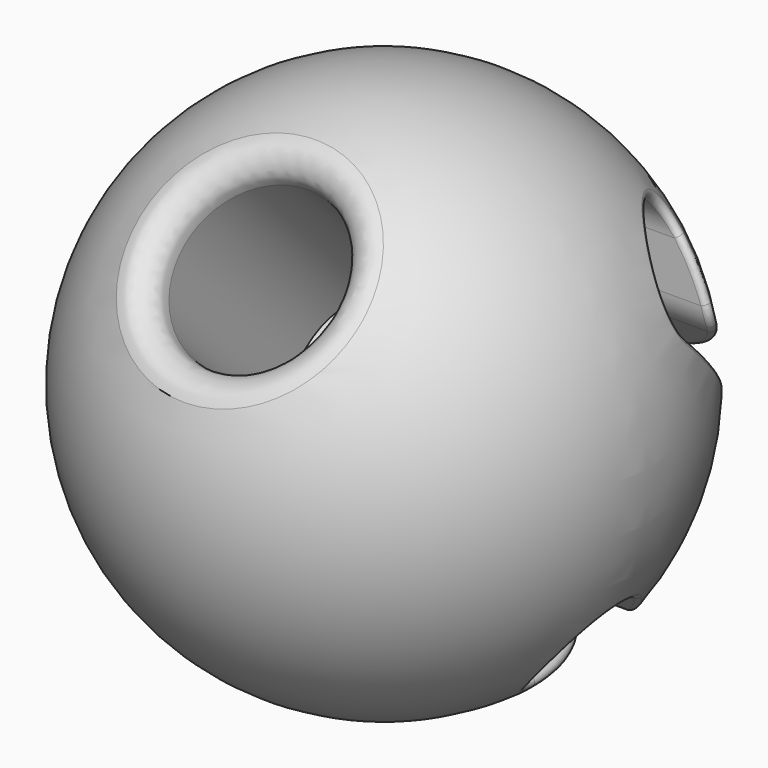
from build123d import *

# Parameters (mm, degrees)
F5_R     = 1
F6_DEPTH = 4
F8_DEPTH = 12.5
F9_R     = 0.3
F10_R    = 0.06


with BuildPart() as f2:
    # F0 (on Front) → F2 (revolve)
    with BuildSketch(Plane.XZ):
        with BuildLine():
            ThreePointArc((0, -3.25), (3.25, 0), (0, 3.25))
            Line((0, 3.25), (0, -3.25))
        make_face()
    revolve(axis=Axis((0, 0, 0.1662829891), (0, 0, 1)))

    # F5 (on face) → F6 (cut)
    with BuildSketch(Plane(origin=(0, -2.8284271247, 2.8284271247), x_dir=(1, 0, 0), z_dir=(0, -0.7071067812, 0.7071067812))):
        Circle(F5_R)
    extrude(amount=-F6_DEPTH, mode=Mode.SUBTRACT)

    # F7 (on Right) → F8 (cut, symmetric)
    with BuildSketch(Plane.YZ):
        with BuildLine():
            ThreePointArc((0.4024877285, -1.5893558372), (-0.5323276217, -1.782624051), (0, -2.575))
            Line((0, -2.575), (3.8884331007, -2.575))
            Line((3.8884331007, -2.575), (3.8884331007, -2.175))
            Line((3.8884331007, -2.175), (1.2041749668, -2.175))
            ThreePointArc((1.2041749668, -2.175), (1.0151524025, -2.1378935841), (0.8541856377, -2.0320818807))
            Line((0.8541856377, -2.0320818807), (0.4024877285, -1.5893558372))
        make_face()
        with BuildLine():
            ThreePointArc((1.9891846367, 1.4199810324), (1.1915090989, 1.9443340411), (1.0076271632, 1.0076271632))
            Line((1.0076271632, 1.0076271632), (4.0254975232, -2.0102431969))
            Line((4.0254975232, -2.0102431969), (4.3083402357, -1.7274004844))
            Line((4.3083402357, -1.7274004844), (2.1419501604, 0.4389895909))
            ThreePointArc((2.1419501604, 0.4389895909), (2.0345292217, 0.5988869263), (1.9955287038, 0.7875277902))
            Line((1.9955287038, 0.7875277902), (1.9891846367, 1.4199810324))
        make_face()
    extrude(amount=F8_DEPTH, both=True, mode=Mode.SUBTRACT)

    # F9
    f9_edges = [f2.edges().sort_by_distance(p)[0] for p in [
        (-1, -2.186607, 2.186607),
    ]]
    fillet(f9_edges, radius=F9_R)

    # F10
    f10_edges = [f2.edges().sort_by_distance(p)[0] for p in [
        (0, 3.192032, -0.611092),
        (0, 1.982896, -2.575),
        (-2.625585, -0.550681, -1.834544),
        (2.889816, 0.223487, -1.470209),
        (2.483546, -0.574778, -2.015968),
        (-2.616356, 0.637389, -1.819592),
        (2.616356, 0.637389, -1.819592),
        (-2.232344, 1.009369, -2.135489),
        (2.232344, 1.009369, -2.135489),
        (0, 2.414928, -2.175),
        (2.332135, 1.172747, 1.936055),
        (-2.332135, 1.172747, 1.936055),
        (-2.313521, 1.992254, 1.114023),
        (2.313521, 1.992254, 1.114023),
        (-2.46227, 2.035925, 0.595597),
        (2.46227, 2.035925, 0.595597),
        (0, 3.073042, -1.057787),
    ]]
    fillet(f10_edges, radius=F10_R)


solid = f2.part
